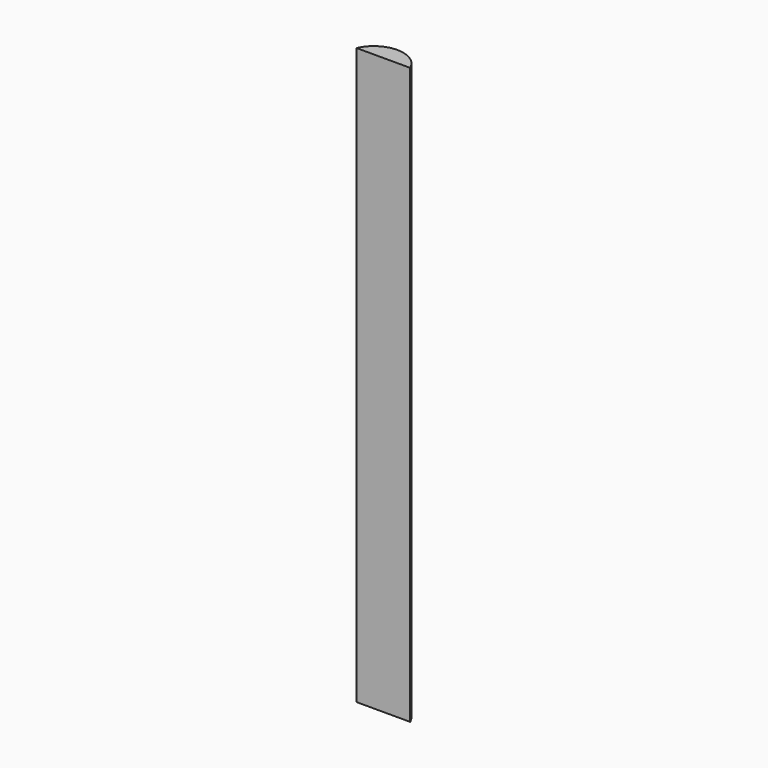
from build123d import *

# Parameters (mm, degrees)
F0_W        = 9.3987649307
F0_H        = 84.1068960726
F1_DEPTH    = 3.048
F2_T1_DEPTH = 107.386380603
F3_DEPTH    = 16.764


# Not quite as in the source:
# - a fillet or chamfer that OpenCascade refuses, or shapes differently, is made with other operations: its cross-section is extruded or revolved along the edge and cut away or added


with BuildPart() as f1:
    # F0 (on Front) → F1 (new body)
    with BuildSketch(Plane.XZ):
        with Locations((-10.7242320664, -3.0124243349)):
            Rectangle(F0_W, F0_H)
    extrude(amount=F1_DEPTH)

    # F2: fillet of radius 5.08 on 2 edges, made by hand

    # F2_s2 → F2_t1 (cut)
    with BuildSketch(Plane.XY.offset(-56.7056146364)):
        with BuildLine():
            ThreePointArc((-6.0248496011, -3.048), (-7.898315915, -0.8297670652), (-10.6807465072, 0))
            Line((-10.6807465072, 0), (-6.0248496011, 0))
            Line((-6.0248496011, 0), (-6.0248496011, -3.048))
        make_face()
        with BuildLine():
            ThreePointArc((-15.4236145318, -3.048), (-13.5501482178, -0.8297670652), (-10.7677176257, 0))
            Line((-10.7677176257, 0), (-15.4236145318, 0))
            Line((-15.4236145318, 0), (-15.4236145318, -3.048))
        make_face()
    extrude(amount=F2_T1_DEPTH, mode=Mode.SUBTRACT)

    # F3 (add): a face of the model
    f3_faces = [f1.faces().sort_by_distance(p)[0] for p in [
        (-10.7242320664, -1.7873359361, 39.0410237014),
    ]]
    extrude(f3_faces, amount=F3_DEPTH)


solid = f1.part
